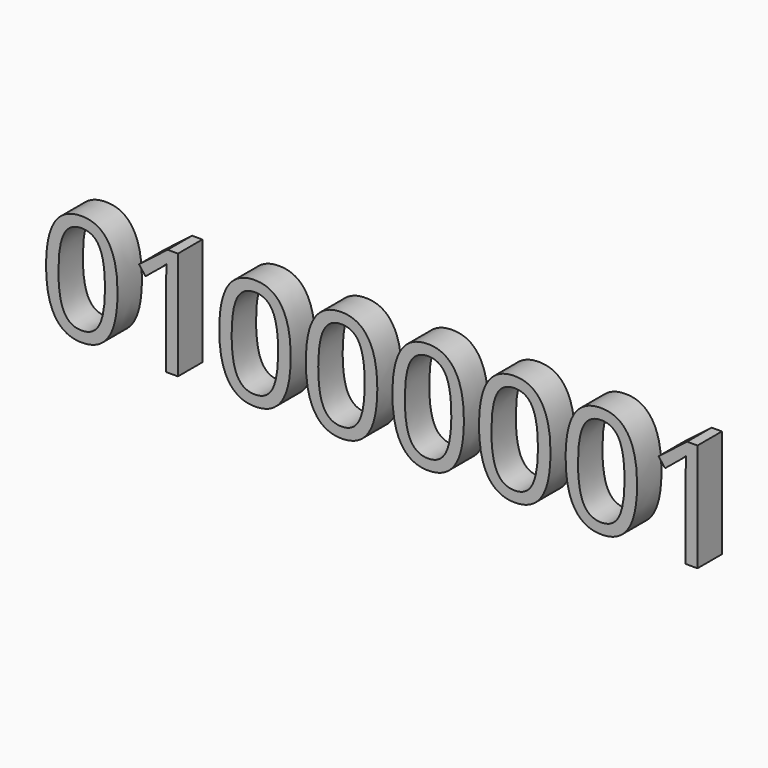
from build123d import *

# Parameters (mm, degrees)
F0_TEXT_SIZE = 125.9964088806
F1_DEPTH     = 25.4


# Not quite as in the source:
# - Text() gives the source's letters only with a copy of the font that has no kerning and outlines rounded to 1/6400 em; it was checked with that copy


with BuildPart() as f1:
    # F0 (on Front) → F1 (new body)
    with BuildSketch(Plane.XZ):
        with Locations((-45.9112264216, -64.1351565719)):
            Text('01000001', F0_TEXT_SIZE, font='Open Sans', text_align=(TextAlign.LEFT, TextAlign.BOTTOM))
    extrude(amount=F1_DEPTH)


solid = f1.part
